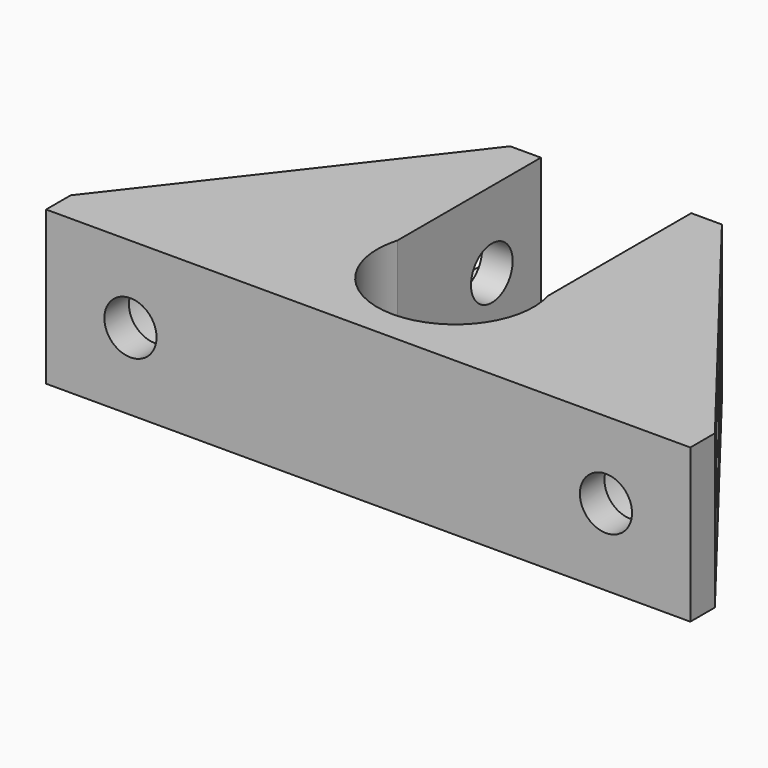
from build123d import *

# Parameters (mm, degrees)
F1_DEPTH      = 5
F2_R          = 1.7
F3_DEPTH      = 20.201
F5_R          = 3
F6_DEPTH      = 18.201
F7_R          = 1.7
F9_DEPTH      = 21.001
F9_DEPTH_BACK = 21.001
F11_DEPTH     = 14.101


# Not quite as in the source:
# - a pattern or mirror of a feature is missing from the dataset's text; its kind, count and spacing are read off the source's solid


with BuildPart() as f1:
    # F0 (on Top) → F1 (new body, symmetric)
    with BuildSketch(Plane.XY):
        with BuildLine():
            Line((-21, 2), (-21, 0))
            Line((-21, 0), (21, 0))
            Line((21, 0), (21, 2))
            Line((21, 2), (6.9, 20.2))
            Line((6.9, 20.2), (4.9, 20.2))
            Line((4.9, 20.2), (4.9, 8.5142135624))
            ThreePointArc((4.9, 8.5142135624), (0, 2), (-4.9, 8.5142135624))
            Line((-4.9, 8.5142135624), (-4.9, 20.2))
            Line((-4.9, 20.2), (-6.9, 20.2))
            Line((-6.9, 20.2), (-21, 2))
        make_face()
    extrude(amount=F1_DEPTH, both=True)

    # F2 (on Front) → F3 (cut, through all)
    with BuildSketch(Plane.XZ):
        with Locations((-15.5, 0)):
            Circle(F2_R)
        with Locations((15.5, 0)):
            Circle(F2_R)
    extrude(amount=-F3_DEPTH, mode=Mode.SUBTRACT)

    # F5 (on plane+point) → F6 (cut, through all)
    with BuildSketch(Plane.XZ.offset(-2)):
        with Locations((-15.5, 0)):
            Circle(F5_R)
        with Locations((15.5, 0)):
            Circle(F5_R)
    extrude(amount=-F6_DEPTH, mode=Mode.SUBTRACT)

    # F7 (on Right) → F9 (cut, two sides)
    with BuildSketch(Plane.YZ) as f9_sk:
        with Locations((16.2, 0)):
            Circle(F7_R)
    extrude(amount=-F9_DEPTH, mode=Mode.SUBTRACT)
    extrude(f9_sk.sketch, amount=F9_DEPTH_BACK, mode=Mode.SUBTRACT)

    # F10 (on plane+point) → F11 (cut, through all)
    with BuildSketch(Plane.YZ.offset(6.9)):
        Polygon((16.2, -3.2908965344), (19.05, -1.6454482672), (19.05, 1.6454482672), (16.2, 3.2908965344), (13.35, 1.6454482672), (13.35, -1.6454482672), align=None)
    f11 = extrude(amount=F11_DEPTH, mode=Mode.SUBTRACT)

    # F11_copies: F11 across plane
    add(f11.mirror(Plane(origin=(0, 0, 0), x_dir=(0, 0, -1), z_dir=(-1, 0, 0))), mode=Mode.SUBTRACT)


solid = f1.part
